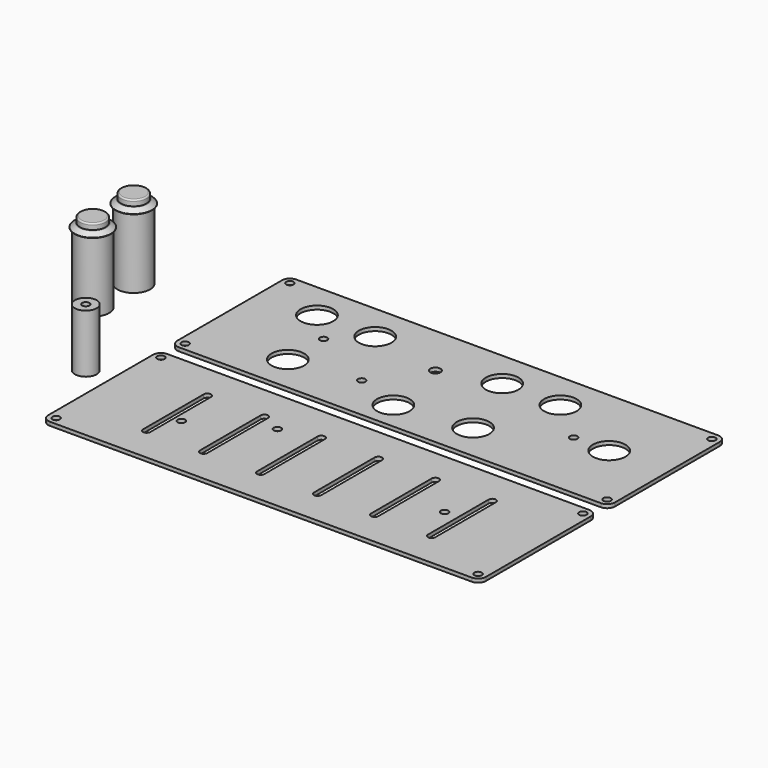
from build123d import *

# Parameters (mm, degrees)
F1_R     = 3.2385
F1_R_2   = 14.25
F1_R_3   = 4.445
F2_DEPTH = 3.175
F3_R     = 9.525
F3_R_2   = 3.175
F4_DEPTH = 50.8
F5_W     = 14.25
F5_H     = 61.19
F5_W_2   = 11.1813665285
F5_H_2   = 5.08
F7_R     = 1.27
F8_R     = 0.254


# Not quite as in the source:
# - a length typed as a fraction of an inch, garbled in the dataset ("3 / 203.2 mm" for 3/8 in), is restored


with BuildPart() as f2:
    # F1 (on Top) → F2 (new body)
    with BuildSketch(Plane.XY):
        with BuildLine():
            Line((264.5218431592, 131.4419915089), (-103.7781568408, 131.4419915089))
            ThreePointArc((-103.7781568408, 131.4419915089), (-108.6454556584, 129.4258903265), (-110.6615568408, 124.5585915089))
            Line((-110.6615568408, 124.5585915089), (-110.6615568408, 10.2585915089))
            ThreePointArc((-110.6615568408, 10.2585915089), (-108.6454556584, 5.3912926912), (-103.7781568408, 3.3751915089))
            Line((-103.7781568408, 3.3751915089), (264.5218431592, 3.3751915089))
            ThreePointArc((264.5218431592, 3.3751915089), (269.3891419768, 5.3912926912), (271.4052431592, 10.2585915089))
            Line((271.4052431592, 10.2585915089), (271.4052431592, 124.5585915089))
            ThreePointArc((271.4052431592, 124.5585915089), (269.3891419768, 129.4258903265), (264.5218431592, 131.4419915089))
        make_face()
        with Locations((-103.7781568408, 10.2585915089)):
            Circle(F1_R, mode=Mode.SUBTRACT)
        with Locations((-34.4615568408, 35.6585915089)):
            Circle(F1_R_2, mode=Mode.SUBTRACT)
        with Locations((63.7149438262, 28.0295349658)):
            Circle(F1_R_2, mode=Mode.SUBTRACT)
        with Locations((24.1264589131, 43.005399406)):
            Circle(F1_R, mode=Mode.SUBTRACT)
        with Locations((-34.4615568408, 74.599519372)):
            Circle(F1_R, mode=Mode.SUBTRACT)
        with Locations((-103.7781568408, 124.5585915089)):
            Circle(F1_R, mode=Mode.SUBTRACT)
        with Locations((-59.8615568408, 99.1585915089)):
            Circle(F1_R_2, mode=Mode.SUBTRACT)
        with Locations((54.2252957821, 85.7786983252)):
            Circle(F1_R_3, mode=Mode.SUBTRACT)
        with Locations((-9.0615568408, 99.1585915089)):
            Circle(F1_R_2, mode=Mode.SUBTRACT)
        with Locations((127.2149438262, 35.6585915089)):
            Circle(F1_R_2, mode=Mode.SUBTRACT)
        with Locations((264.5218431592, 10.2585915089)):
            Circle(F1_R, mode=Mode.SUBTRACT)
        with Locations((101.8149438262, 99.1585915089)):
            Circle(F1_R_2, mode=Mode.SUBTRACT)
        with Locations((152.6149438262, 99.1585915089)):
            Circle(F1_R_2, mode=Mode.SUBTRACT)
        with Locations((189.5859390497, 67.4085915089)):
            Circle(F1_R, mode=Mode.SUBTRACT)
        with Locations((220.6052431592, 67.4085915089)):
            Circle(F1_R_2, mode=Mode.SUBTRACT)
        with Locations((264.5218431592, 124.5585915089)):
            Circle(F1_R, mode=Mode.SUBTRACT)
    extrude(amount=-F2_DEPTH)


with BuildPart() as f2b:
    # F1 (on Top) → F2, piece 2 (new body)
    with BuildSketch(Plane.XY):
        with BuildLine():
            ThreePointArc((-110.6615568408, -130.5082084911), (-108.6454556584, -135.3755073088), (-103.7781568408, -137.3916084911))
            Line((-103.7781568408, -137.3916084911), (264.5218431592, -137.3916084911))
            ThreePointArc((264.5218431592, -137.3916084911), (269.3891419768, -135.3755073088), (271.4052431592, -130.5082084911))
            Line((271.4052431592, -130.5082084911), (271.4052431592, -16.2082084911))
            ThreePointArc((271.4052431592, -16.2082084911), (269.3891419768, -11.3409096735), (264.5218431592, -9.3248084911))
            Line((264.5218431592, -9.3248084911), (-103.7781568408, -9.3248084911))
            ThreePointArc((-103.7781568408, -9.3248084911), (-108.6454556584, -11.3409096735), (-110.6615568408, -16.2082084911))
            Line((-110.6615568408, -16.2082084911), (-110.6615568408, -130.5082084911))
        make_face()
        with Locations((-103.7781568408, -130.5082084911)):
            Circle(F1_R, mode=Mode.SUBTRACT)
        with BuildLine():
            Line((-47.1615568408, -106.4528019969), (-47.1615568408, -40.2636149853))
            ThreePointArc((-47.1615568408, -40.2636149853), (-43.9865568408, -37.0886149853), (-40.8115568408, -40.2636149853))
            Line((-40.8115568408, -40.2636149853), (-40.8115568408, -106.4528019969))
            ThreePointArc((-40.8115568408, -106.4528019969), (-43.9865568408, -109.6278019969), (-47.1615568408, -106.4528019969))
        make_face(mode=Mode.SUBTRACT)
        with Locations((-34.4615568408, -80.5491363543)):
            Circle(F1_R, mode=Mode.SUBTRACT)
        with BuildLine():
            ThreePointArc((2.5818031592, -40.2636149853), (5.7568031592, -37.0886149853), (8.9318031592, -40.2636149853))
            Line((8.9318031592, -40.2636149853), (8.9318031592, -106.4528019969))
            ThreePointArc((8.9318031592, -106.4528019969), (5.7568031592, -109.6278019969), (2.5818031592, -106.4528019969))
            Line((2.5818031592, -106.4528019969), (2.5818031592, -40.2636149853))
        make_face(mode=Mode.SUBTRACT)
        with BuildLine():
            ThreePointArc((52.3251631592, -40.2636149853), (55.5001631592, -37.0886149853), (58.6751631592, -40.2636149853))
            Line((58.6751631592, -40.2636149853), (58.6751631592, -106.4528019969))
            ThreePointArc((58.6751631592, -106.4528019969), (55.5001631592, -109.6278019969), (52.3251631592, -106.4528019969))
            Line((52.3251631592, -106.4528019969), (52.3251631592, -40.2636149853))
        make_face(mode=Mode.SUBTRACT)
        with Locations((-103.7781568408, -16.2082084911)):
            Circle(F1_R, mode=Mode.SUBTRACT)
        with Locations((24.1264589131, -48.9550163882)):
            Circle(F1_R, mode=Mode.SUBTRACT)
        with BuildLine():
            ThreePointArc((102.0685231592, -40.2636149853), (105.2435231592, -37.0886149853), (108.4185231592, -40.2636149853))
            Line((108.4185231592, -40.2636149853), (108.4185231592, -106.4528019969))
            ThreePointArc((108.4185231592, -106.4528019969), (105.2435231592, -109.6278019969), (102.0685231592, -106.4528019969))
            Line((102.0685231592, -106.4528019969), (102.0685231592, -40.2636149853))
        make_face(mode=Mode.SUBTRACT)
        with BuildLine():
            ThreePointArc((151.8118831592, -40.2636149853), (154.9868831592, -37.0886149853), (158.1618831592, -40.2636149853))
            Line((158.1618831592, -40.2636149853), (158.1618831592, -106.4528019969))
            ThreePointArc((158.1618831592, -106.4528019969), (154.9868831592, -109.6278019969), (151.8118831592, -106.4528019969))
            Line((151.8118831592, -106.4528019969), (151.8118831592, -40.2636149853))
        make_face(mode=Mode.SUBTRACT)
        with Locations((264.5218431592, -130.5082084911)):
            Circle(F1_R, mode=Mode.SUBTRACT)
        with Locations((189.5859390497, -73.3582084911)):
            Circle(F1_R, mode=Mode.SUBTRACT)
        with BuildLine():
            ThreePointArc((201.5552431592, -40.2636149853), (204.7302431592, -37.0886149853), (207.9052431592, -40.2636149853))
            Line((207.9052431592, -40.2636149853), (207.9052431592, -106.4528019969))
            ThreePointArc((207.9052431592, -106.4528019969), (204.7302431592, -109.6278019969), (201.5552431592, -106.4528019969))
            Line((201.5552431592, -106.4528019969), (201.5552431592, -40.2636149853))
        make_face(mode=Mode.SUBTRACT)
        with Locations((264.5218431592, -16.2082084911)):
            Circle(F1_R, mode=Mode.SUBTRACT)
    extrude(amount=-F2_DEPTH)


with BuildPart() as f4:
    # F3 (on Top) → F4 (new body)
    with BuildSketch(Plane.XY):
        with Locations((-132.05742836, -62.824614346)):
            Circle(F3_R)
        with Locations((-132.05742836, -62.824614346)):
            Circle(F3_R_2, mode=Mode.SUBTRACT)
    extrude(amount=F4_DEPTH)


with BuildPart() as f6:
    # F5 (on Front) → F6 (revolve)
    with BuildSketch(Plane.XZ):
        with BuildLine():
            Line((-165.0554220757, 73.7161731559), (-176.2367886041, 73.7161731559))
            Line((-176.2367886041, 73.7161731559), (-176.2367886041, 69.9061731559))
            Line((-176.2367886041, 69.9061731559), (-161.9867886041, 69.9061731559))
            Line((-161.9867886041, 69.9061731559), (-159.8367886041, 69.9061731559))
            Line((-159.8367886041, 69.9061731559), (-164.2632241513, 73.4388072519))
            ThreePointArc((-164.2632241513, 73.4388072519), (-164.6357467857, 73.6448276728), (-165.0554220757, 73.7161731559))
        make_face()
        with Locations((-169.1117886041, 39.3111731559)):
            Rectangle(F5_W, F5_H)
        with Locations((-170.6461053399, 76.2561731559)):
            Rectangle(F5_W_2, F5_H_2)
    revolve(axis=Axis((-176.2367886041, 0, 41.2161731559), (0, 0, -1)))

    # F7
    f7_edges = [f6.edges().sort_by_distance(p)[0] for p in [
        (-187.418155, 0, 78.796173),
    ]]
    fillet(f7_edges, radius=F7_R)

    # F8
    f8_edges = [f6.edges().sort_by_distance(p)[0] for p in [
        (-192.636789, 0, 69.906173),
    ]]
    fillet(f8_edges, radius=F8_R)


with BuildPart() as f9_1:
    # F9: copy of F6
    add(f6.part.moved(Location((0, 44.704, 0))))


solid = Compound([f2.part, f2b.part, f4.part, f6.part, f9_1.part])
